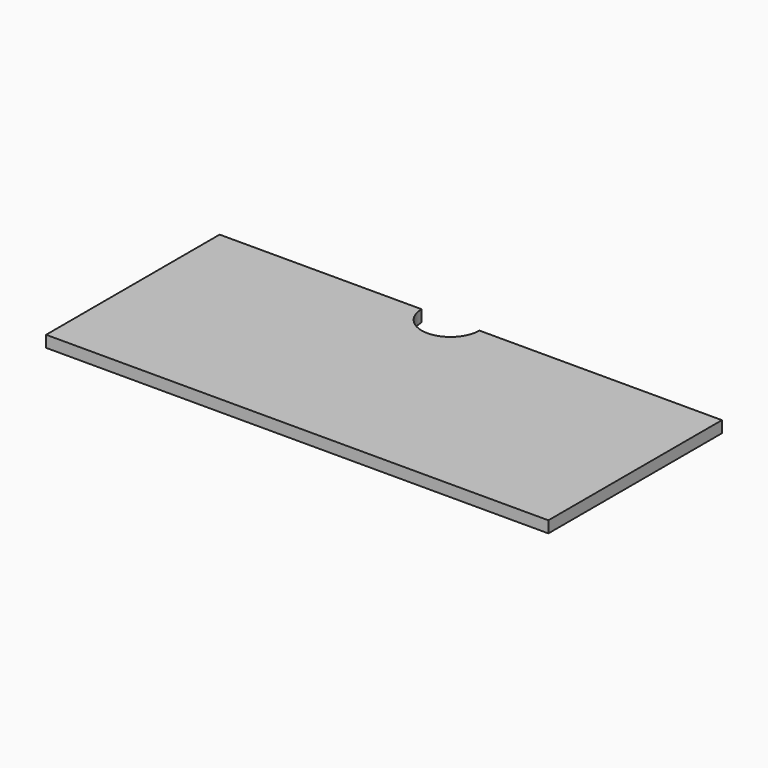
from build123d import *

# Parameters (mm, degrees)
F1_DEPTH = 2


with BuildPart() as f1:
    # F0 (on Top) → F1 (new body)
    with BuildSketch(Plane.XY):
        with BuildLine():
            Line((35, 0), (5, 0))
            ThreePointArc((5, 0), (0, -5), (-5, 0))
            Line((-5, 0), (-35, 0))
            ThreePointArc((-35, 0), (0, -35), (35, 0))
        make_face()
        with BuildLine():
            Line((47, 0), (35, 0))
            ThreePointArc((35, 0), (0, -35), (-35, 0))
            Line((-35, 0), (-40, 0))
            Line((-40, 0), (-40, -37.5692024827))
            Line((-40, -37.5692024827), (47, -37.5692024827))
            Line((47, -37.5692024827), (47, 0))
        make_face()
    extrude(amount=F1_DEPTH)


solid = f1.part
